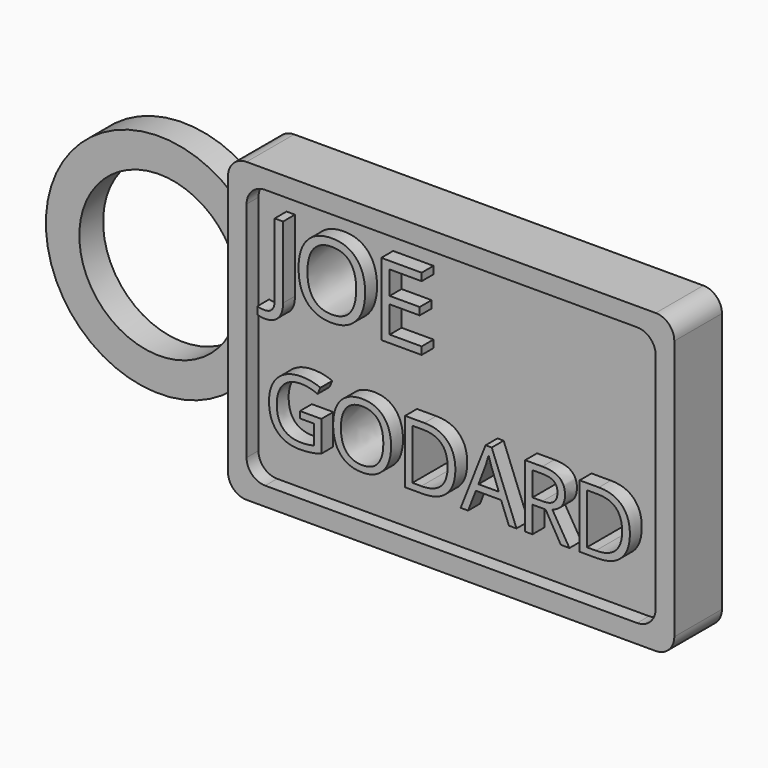
from build123d import *

# Parameters (mm, degrees)
F1_DEPTH       = 20.32
F2_DEPTH       = 15.24
F0_R           = 27.2915133995
F3_DEPTH       = 10.16
F0_TEXT_SIZE   = 34.6307746238
F0_TEXT_SIZE_2 = 30.0981299759
F4_DEPTH       = 20.32


# Not quite as in the source:
# - Text() gives the source's letters only with a copy of the font that has no kerning and outlines rounded to 1/6400 em; it was checked with that copy


with BuildPart() as f1:
    # F0 (on Front) → F1 (new body)
    with BuildSketch(Plane.XZ):
        with BuildLine():
            ThreePointArc((0, 6.35), (1.8598719395, 1.8598719395), (6.35, 0))
            Line((6.35, 0), (146.05, 0))
            ThreePointArc((146.05, 0), (150.5401280605, 1.8598719395), (152.4, 6.35))
            Line((152.4, 6.35), (152.4, 95.25))
            ThreePointArc((152.4, 95.25), (150.5401280605, 99.7401280605), (146.05, 101.6))
            Line((146.05, 101.6), (6.35, 101.6))
            ThreePointArc((6.35, 101.6), (1.8598719395, 99.7401280605), (0, 95.25))
            Line((0, 95.25), (0, 76.4830120565))
            Line((0, 76.4830120565), (0, 31.7811063765))
            Line((0, 31.7811063765), (0, 6.35))
        make_face()
        with BuildLine():
            ThreePointArc((6.35, 88.9), (8.2098719395, 93.3901280605), (12.7, 95.25))
            Line((12.7, 95.25), (139.7, 95.25))
            ThreePointArc((139.7, 95.25), (144.1901280605, 93.3901280605), (146.05, 88.9))
            Line((146.05, 88.9), (146.05, 12.7))
            ThreePointArc((146.05, 12.7), (144.1901280605, 8.2098719395), (139.7, 6.35))
            Line((139.7, 6.35), (12.7, 6.35))
            ThreePointArc((12.7, 6.35), (8.2098719395, 8.2098719395), (6.35, 12.7))
            Line((6.35, 12.7), (6.35, 88.9))
        make_face(mode=Mode.SUBTRACT)
    extrude(amount=F1_DEPTH)

    # F0 (on Front) → F2 (join)
    with BuildSketch(Plane.XZ):
        with BuildLine():
            Line((139.7, 95.25), (12.7, 95.25))
            ThreePointArc((12.7, 95.25), (8.2098719395, 93.3901280605), (6.35, 88.9))
            Line((6.35, 88.9), (6.35, 12.7))
            ThreePointArc((6.35, 12.7), (8.2098719395, 8.2098719395), (12.7, 6.35))
            Line((12.7, 6.35), (139.7, 6.35))
            ThreePointArc((139.7, 6.35), (144.1901280605, 8.2098719395), (146.05, 12.7))
            Line((146.05, 12.7), (146.05, 88.9))
            ThreePointArc((146.05, 88.9), (144.1901280605, 93.3901280605), (139.7, 95.25))
        make_face()
        with BuildLine():
            Line((24.5773977576, 30.4042935003), (24.5773977576, 32.6381390844))
            Line((24.5773977576, 32.6381390844), (31.8808971096, 32.6381390844))
            Line((31.8808971096, 32.6381390844), (31.8808971096, 22.1884445834))
            add(Edge.make_bspline(
                [(31.8808971096, 22.1884445834), (30.1737688, 21.6429159776), (28.4102064967, 21.3630974255)],
                knots=[0, 0, 0, 1, 1, 1], degree=2))
            add(Edge.make_bspline(
                [(28.4102064967, 21.3630974255), (26.6466441934, 21.0832788733), (24.3234447859, 21.0832788733)],
                knots=[0, 0, 0, 1, 1, 1], degree=2))
            add(Edge.make_bspline(
                [(24.3234447859, 21.0832788733), (19.4466071633, 21.0832788733), (16.7283697998, 23.9872781327)],
                knots=[0, 0, 0, 1, 1, 1], degree=2))
            add(Edge.make_bspline(
                [(16.7283697998, 23.9872781327), (14.0101324364, 26.8912773921), (14.0101324364, 32.1208274754)],
                knots=[0, 0, 0, 1, 1, 1], degree=2))
            add(Edge.make_bspline(
                [(14.0101324364, 32.1208274754), (14.0101324364, 35.4739472681), (15.3551426197, 37.9946656536)],
                knots=[0, 0, 0, 1, 1, 1], degree=2))
            add(Edge.make_bspline(
                [(15.3551426197, 37.9946656536), (16.700152803, 40.515384039), (19.2279254377, 41.8439343075)],
                knots=[0, 0, 0, 1, 1, 1], degree=2))
            add(Edge.make_bspline(
                [(19.2279254377, 41.8439343075), (21.7556980724, 43.172484576), (25.1464405275, 43.172484576)],
                knots=[0, 0, 0, 1, 1, 1], degree=2))
            add(Edge.make_bspline(
                [(25.1464405275, 43.172484576), (28.5889141435, 43.172484576), (31.5564016458, 41.9121253832)],
                knots=[0, 0, 0, 1, 1, 1], degree=2))
            Line((31.5564016458, 41.9121253832), (30.5876180872, 39.7064967959))
            add(Edge.make_bspline(
                [(30.5876180872, 39.7064967959), (27.6765645786, 40.9386389918), (24.986544212, 40.9386389918)],
                knots=[0, 0, 0, 1, 1, 1], degree=2))
            add(Edge.make_bspline(
                [(24.986544212, 40.9386389918), (21.0643816495, 40.9386389918), (18.8587530622, 38.6036825023)],
                knots=[0, 0, 0, 1, 1, 1], degree=2))
            add(Edge.make_bspline(
                [(18.8587530622, 38.6036825023), (16.6531244749, 36.2687260128), (16.6531244749, 32.1208274754)],
                knots=[0, 0, 0, 1, 1, 1], degree=2))
            add(Edge.make_bspline(
                [(16.6531244749, 32.1208274754), (16.6531244749, 27.7707071274), (18.776453488, 25.5227530448)],
                knots=[0, 0, 0, 1, 1, 1], degree=2))
            add(Edge.make_bspline(
                [(18.776453488, 25.5227530448), (20.8997825012, 23.2747989622), (25.0147612088, 23.2747989622)],
                knots=[0, 0, 0, 1, 1, 1], degree=2))
            add(Edge.make_bspline(
                [(25.0147612088, 23.2747989622), (27.248606793, 23.2747989622), (29.3789900553, 23.7921105712)],
                knots=[0, 0, 0, 1, 1, 1], degree=2))
            Line((29.3789900553, 23.7921105712), (29.3789900553, 30.4042935003))
            Line((29.3789900553, 30.4042935003), (24.5773977576, 30.4042935003))
        make_face(mode=Mode.SUBTRACT)
        with BuildLine():
            add(Edge.make_bspline(
                [(53.0859702442, 40.2661339002), (55.6866367874, 37.3268633947), (55.6866367874, 32.1537473051)],
                knots=[0, 0, 0, 1, 1, 1], degree=2))
            add(Edge.make_bspline(
                [(55.6866367874, 32.1537473051), (55.6866367874, 26.9947397139), (53.0765645786, 24.0390092936)],
                knots=[0, 0, 0, 1, 1, 1], degree=2))
            add(Edge.make_bspline(
                [(53.0765645786, 24.0390092936), (50.4664923697, 21.0832788733), (45.8247963875, 21.0832788733)],
                knots=[0, 0, 0, 1, 1, 1], degree=2))
            add(Edge.make_bspline(
                [(45.8247963875, 21.0832788733), (41.0796380835, 21.0832788733), (38.5001342879, 23.9872781327)],
                knots=[0, 0, 0, 1, 1, 1], degree=2))
            add(Edge.make_bspline(
                [(38.5001342879, 23.9872781327), (35.9206304923, 26.8912773921), (35.9206304923, 32.181964302)],
                knots=[0, 0, 0, 1, 1, 1], degree=2))
            add(Edge.make_bspline(
                [(35.9206304923, 32.181964302), (35.9206304923, 37.4303257165), (38.5071885371, 40.3178650611)],
                knots=[0, 0, 0, 1, 1, 1], degree=2))
            add(Edge.make_bspline(
                [(38.5071885371, 40.3178650611), (41.0937465819, 43.2054044056), (45.8530133843, 43.2054044056)],
                knots=[0, 0, 0, 1, 1, 1], degree=2))
            add(Edge.make_bspline(
                [(45.8530133843, 43.2054044056), (50.4853037009, 43.2054044056), (53.0859702442, 40.2661339002)],
                knots=[0, 0, 0, 1, 1, 1], degree=2))
        make_face(mode=Mode.SUBTRACT)
        with BuildLine():
            add(Edge.make_bspline(
                [(74.8483290666, 40.0897776699), (77.6253518402, 37.3127548963), (77.6253518402, 32.327752119)],
                knots=[0, 0, 0, 1, 1, 1], degree=2))
            add(Edge.make_bspline(
                [(77.6253518402, 32.327752119), (77.6253518402, 27.0088482123), (74.7378124956, 24.1942027763)],
                knots=[0, 0, 0, 1, 1, 1], degree=2))
            add(Edge.make_bspline(
                [(74.7378124956, 24.1942027763), (71.850273151, 21.3795573403), (66.4279069226, 21.3795573403)],
                knots=[0, 0, 0, 1, 1, 1], degree=2))
            Line((66.4279069226, 21.3795573403), (60.4741205867, 21.3795573403))
            Line((60.4741205867, 21.3795573403), (60.4741205867, 42.8668004434))
            Line((60.4741205867, 42.8668004434), (67.0580865189, 42.8668004434))
            add(Edge.make_bspline(
                [(67.0580865189, 42.8668004434), (72.0713062931, 42.8668004434), (74.8483290666, 40.0897776699)],
                knots=[0, 0, 0, 1, 1, 1], degree=2))
        make_face(mode=Mode.SUBTRACT)
        Polygon((98.5106323438, 21.3795573403), (95.924074299, 21.3795573403), (93.2481624308, 28.2127734114), (84.637275558, 28.2127734114), (81.9942835195, 21.3795573403), (79.4641594684, 21.3795573403), (87.957475521, 42.9561542668), (90.0596417865, 42.9561542668), align=None, mode=Mode.SUBTRACT)
        with BuildLine():
            Line((108.4477180687, 30.3149396769), (103.9612155691, 30.3149396769))
            Line((103.9612155691, 30.3149396769), (103.9612155691, 21.3795573403))
            Line((103.9612155691, 21.3795573403), (101.4640113477, 21.3795573403))
            Line((101.4640113477, 21.3795573403), (101.4640113477, 42.8668004434))
            Line((101.4640113477, 42.8668004434), (107.356660857, 42.8668004434))
            add(Edge.make_bspline(
                [(107.356660857, 42.8668004434), (111.3117432492, 42.8668004434), (113.1999306219, 41.352488279)],
                knots=[0, 0, 0, 1, 1, 1], degree=2))
            add(Edge.make_bspline(
                [(113.1999306219, 41.352488279), (115.0881179946, 39.8381761146), (115.0881179946, 36.7954432873)],
                knots=[0, 0, 0, 1, 1, 1], degree=2))
            add(Edge.make_bspline(
                [(115.0881179946, 36.7954432873), (115.0881179946, 32.5346767626), (110.7662146434, 31.0344730966)],
                knots=[0, 0, 0, 1, 1, 1], degree=2))
            Line((110.7662146434, 31.0344730966), (116.602430159, 21.3795573403))
            Line((116.602430159, 21.3795573403), (113.6490511551, 21.3795573403))
            Line((113.6490511551, 21.3795573403), (108.4477180687, 30.3149396769))
        make_face(mode=Mode.SUBTRACT)
        with BuildLine():
            add(Edge.make_bspline(
                [(134.442626419, 40.0897776699), (137.2196491925, 37.3127548963), (137.2196491925, 32.327752119)],
                knots=[0, 0, 0, 1, 1, 1], degree=2))
            add(Edge.make_bspline(
                [(137.2196491925, 32.327752119), (137.2196491925, 27.0088482123), (134.332109848, 24.1942027763)],
                knots=[0, 0, 0, 1, 1, 1], degree=2))
            add(Edge.make_bspline(
                [(134.332109848, 24.1942027763), (131.4445705034, 21.3795573403), (126.0222042749, 21.3795573403)],
                knots=[0, 0, 0, 1, 1, 1], degree=2))
            Line((126.0222042749, 21.3795573403), (120.0684179391, 21.3795573403))
            Line((120.0684179391, 21.3795573403), (120.0684179391, 42.8668004434))
            Line((120.0684179391, 42.8668004434), (126.6523838713, 42.8668004434))
            add(Edge.make_bspline(
                [(126.6523838713, 42.8668004434), (131.6656036454, 42.8668004434), (134.442626419, 40.0897776699)],
                knots=[0, 0, 0, 1, 1, 1], degree=2))
        make_face(mode=Mode.SUBTRACT)
        with BuildLine():
            add(Edge.make_bspline(
                [(17.1895407936, 58.2547495158), (15.5662232331, 56.4880389041), (12.5197972779, 56.4880389041)],
                knots=[0, 0, 0, 1, 1, 1], degree=2))
            add(Edge.make_bspline(
                [(12.5197972779, 56.4880389041), (10.9343571271, 56.4880389041), (10.0198882347, 56.942567821)],
                knots=[0, 0, 0, 1, 1, 1], degree=2))
            Line((10.0198882347, 56.942567821), (10.0198882347, 59.3937773374))
            add(Edge.make_bspline(
                [(10.0198882347, 59.3937773374), (11.2211432295, 59.0582917082), (12.5197972779, 59.0582917082)],
                knots=[0, 0, 0, 1, 1, 1], degree=2))
            add(Edge.make_bspline(
                [(12.5197972779, 59.0582917082), (14.1972254237, 59.0582917082), (15.0684058479, 60.0728651835)],
                knots=[0, 0, 0, 1, 1, 1], degree=2))
            add(Edge.make_bspline(
                [(15.0684058479, 60.0728651835), (15.939586272, 61.0874386588), (15.939586272, 62.9975423217)],
                knots=[0, 0, 0, 1, 1, 1], degree=2))
            Line((15.939586272, 62.9975423217), (15.939586272, 87.720668768))
            Line((15.939586272, 87.720668768), (18.8128583541, 87.720668768))
            Line((18.8128583541, 87.720668768), (18.8128583541, 63.2356288972))
            add(Edge.make_bspline(
                [(18.8128583541, 63.2356288972), (18.8128583541, 60.0214601274), (17.1895407936, 58.2547495158)],
                knots=[0, 0, 0, 1, 1, 1], degree=2))
        make_face(mode=Mode.SUBTRACT)
        with BuildLine():
            add(Edge.make_bspline(
                [(43.8390040783, 84.7283533981), (46.8313194482, 81.3464418138), (46.8313194482, 75.3942774253)],
                knots=[0, 0, 0, 1, 1, 1], degree=2))
            add(Edge.make_bspline(
                [(46.8313194482, 75.3942774253), (46.8313194482, 69.4583462124), (43.8281819612, 66.0574959232)],
                knots=[0, 0, 0, 1, 1, 1], degree=2))
            add(Edge.make_bspline(
                [(43.8281819612, 66.0574959232), (40.8250444743, 62.656645634), (35.4843297003, 62.656645634)],
                knots=[0, 0, 0, 1, 1, 1], degree=2))
            add(Edge.make_bspline(
                [(35.4843297003, 62.656645634), (30.0245716385, 62.656645634), (27.0566060321, 65.9979742793)],
                knots=[0, 0, 0, 1, 1, 1], degree=2))
            add(Edge.make_bspline(
                [(27.0566060321, 65.9979742793), (24.0886404257, 69.3393029247), (24.0886404257, 75.4267437765)],
                knots=[0, 0, 0, 1, 1, 1], degree=2))
            add(Edge.make_bspline(
                [(24.0886404257, 75.4267437765), (24.0886404257, 81.4654851015), (27.0647226199, 84.787875042)],
                knots=[0, 0, 0, 1, 1, 1], degree=2))
            add(Edge.make_bspline(
                [(27.0647226199, 84.787875042), (30.0408048141, 88.1102649825), (35.5167960515, 88.1102649825)],
                knots=[0, 0, 0, 1, 1, 1], degree=2))
            add(Edge.make_bspline(
                [(35.5167960515, 88.1102649825), (40.8466887085, 88.1102649825), (43.8390040783, 84.7283533981)],
                knots=[0, 0, 0, 1, 1, 1], degree=2))
        make_face(mode=Mode.SUBTRACT)
        Polygon((66.1217431253, 65.5677951258), (66.1217431253, 62.9975423217), (52.3397770368, 62.9975423217), (52.3397770368, 87.720668768), (66.1217431253, 87.720668768), (66.1217431253, 85.1666491395), (55.2130491188, 85.1666491395), (55.2130491188, 77.201570976), (65.4615939841, 77.201570976), (65.4615939841, 74.6637845231), (55.2130491188, 74.6637845231), (55.2130491188, 65.5677951258), align=None, mode=Mode.SUBTRACT)
    extrude(amount=F2_DEPTH)

    # F0 (on Front) → F3 (join)
    with BuildSketch(Plane.XZ):
        with BuildLine():
            ThreePointArc((0, 76.4830120565), (-70.3092045361, 54.1320592165), (0, 31.7811063765))
            Line((0, 31.7811063765), (0, 76.4830120565))
        make_face()
        with Locations((-31.601972878, 54.1320592165)):
            Circle(F0_R, mode=Mode.SUBTRACT)
    extrude(amount=F3_DEPTH)

    # F0 (on Front) → F4 (join)
    with BuildSketch(Plane.XZ):
        with Locations((12.7254175022, 62.9975423217)):
            Text('JOE', F0_TEXT_SIZE, font='Open Sans', text_align=(TextAlign.LEFT, TextAlign.BOTTOM))
        with Locations((12.1713248082, 21.3795573403)):
            Text('GODARD', F0_TEXT_SIZE_2, font='Open Sans', text_align=(TextAlign.LEFT, TextAlign.BOTTOM))
    extrude(amount=F4_DEPTH)


solid = f1.part
